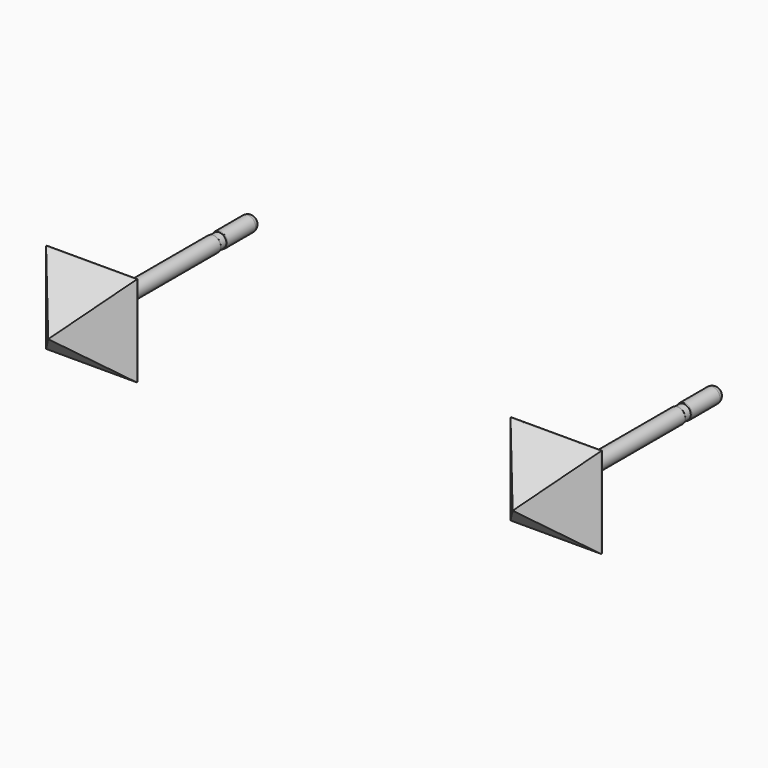
from build123d import *

# Parameters (mm, degrees)
F0_W     = 5.08
F0_H     = 5.08
F2_R     = 0.424942
F3_DEPTH = 10.9982
F4_R     = 0.381
F5_R     = 0.0508
F7_W     = 0.381
F7_H     = 0.1685054609


# Not quite as in the source:
# - a fillet or chamfer that OpenCascade refuses, or shapes differently, is made with other operations: its cross-section is extruded or revolved along the edge and cut away or added
# - an extrude whose draft closes it to a point is written as a loft to that point


with BuildPart() as f1:
    # F0 (on Front) → F1 section 0
    with BuildSketch(Plane.XZ, mode=Mode.PRIVATE) as f1_s0:
        with Locations((12.7, 2.54)):
            Rectangle(F0_W, F0_H)
    loft([f1_s0.sketch, Vertex(12.7, -3.0270541252, 2.54)], ruled=True)

    # F2 (on Front) → F3 (join)
    with BuildSketch(Plane.XZ):
        with Locations((12.7, 2.54)):
            Circle(F2_R)
    extrude(amount=-F3_DEPTH)

    # F4
    f4_edges = [f1.edges().sort_by_distance(p)[0] for p in [
        (12.275058, 10.9982, 2.54),
    ]]
    fillet(f4_edges, radius=F4_R)

    # F5
    f5_edges = [f1.edges().sort_by_distance(p)[0] for p in [
        (15.24, 0, 2.54),
        (12.7, 0, 5.08),
        (10.16, 0, 2.54),
        (12.7, 0, 0),
    ]]
    fillet(f5_edges, radius=F5_R)

    # F7 (on offset) → F8 (revolve, cut)
    with BuildSketch(Plane.YZ.offset(12.7)):
        with Locations((8.4709, 3.0179527304)):
            Rectangle(F7_W, F7_H)
    revolve(axis=Axis((12.7, 9.1875067446, 2.54), (0, 1, 0)), mode=Mode.SUBTRACT)

    # F9: fillet of radius 0.0508 on 2 edges, made by hand

    # F9_s1 → F9_t2 (revolve, cut)
    with BuildSketch(Plane.XY.offset(2.54)):
        with BuildLine():
            ThreePointArc((13.124942, 8.2335158381), (13.1164160251, 8.2616858008), (13.0937, 8.2804))
            Line((13.0937, 8.2804), (13.124942, 8.2804))
            Line((13.124942, 8.2804), (13.124942, 8.2335158381))
        make_face()
    revolve(axis=Axis((12.7, 8.2804, 2.54), (0, -1, 0)), mode=Mode.SUBTRACT)

    # F9_s3 → F9_t4 (revolve, cut)
    with BuildSketch(Plane.XY.offset(2.54)):
        with BuildLine():
            ThreePointArc((13.0937, 8.6614), (13.1164160251, 8.6801141992), (13.124942, 8.7082841619))
            Line((13.124942, 8.7082841619), (13.124942, 8.6614))
            Line((13.124942, 8.6614), (13.0937, 8.6614))
        make_face()
    revolve(axis=Axis((12.7, 8.6614, 2.54), (0, -1, 0)), mode=Mode.SUBTRACT)


with BuildPart() as f10_1:
    # F10: instance of F1
    add(f1.part.mirror(Plane.YZ))


solid = Compound([f1.part, f10_1.part])
